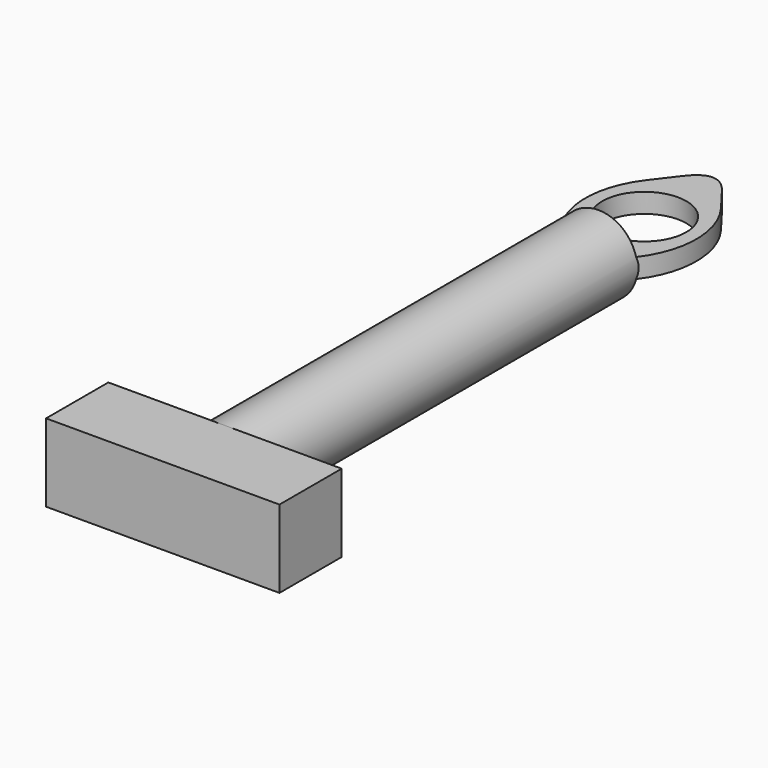
from build123d import *

# Parameters (mm, degrees)
F0_R        = 1.5875
F1_DEPTH    = 25.4
F2_W        = 9.525
F2_H        = 3.175
F3_DEPTH    = 3.175
F5_DEPTH    = 6.35
F7_DEPTH    = 25.4
F8_T1_DEPTH = 7.469008
F10_DEPTH   = 0.79375
F11_R       = 1.7145
F12_DEPTH   = 25.4


# Not quite as in the source:
# - a fillet or chamfer that OpenCascade refuses, or shapes differently, is made with other operations: its cross-section is extruded or revolved along the edge and cut away or added


with BuildPart() as f1:
    # F0 (on Front) → F1 (new body)
    with BuildSketch(Plane.XZ):
        Circle(F0_R)
    extrude(amount=F1_DEPTH)

    # F2 (on face) → F3 (join)
    with BuildSketch(Plane.XZ.offset(25.4)):
        Rectangle(F2_W, F2_H)
    extrude(amount=F3_DEPTH)

    # F4 (on face) → F5 (cut)
    with BuildSketch(Plane(origin=(0, 0, 0), x_dir=(-1, 0, 0), z_dir=(0, 1, 0))):
        with BuildLine():
            Line((-1.53709, 0.396875), (1.53709, 0.396875))
            ThreePointArc((1.53709, 0.396875), (0, 1.5875), (-1.53709, 0.396875))
        make_face()
        with BuildLine():
            Line((1.53709, -0.396875), (-1.53709, -0.396875))
            ThreePointArc((-1.53709, -0.396875), (0, -1.5875), (1.53709, -0.396875))
        make_face()
    extrude(amount=-F5_DEPTH, mode=Mode.SUBTRACT)

    # F6 (on face) → F7 (cut)
    with BuildSketch(Plane(origin=(0, 0, -0.396875), x_dir=(1, 0, 0), z_dir=(0, 0, -1))):
        Polygon((1.53709, 2.019778), (0, 0), (-1.53709, 2.019778), (-2.909934, 3.823732), (-2.909934, -0.784444), (2.909934, -0.784444), (2.909934, 3.823732), align=None)
    extrude(amount=-F7_DEPTH, mode=Mode.SUBTRACT)

    # F8: fillet of radius 1.016 on 1 edges, made by hand

    # F8_s2 → F8_t1 (cut)
    with BuildSketch(Plane.XY.offset(-3.734504)):
        with BuildLine():
            add(Edge.make_bspline(
                [(0.808504, -1.062396), (0, 0), (-0.808504, -1.062396)],
                knots=[0, 0, 0, 1, 1, 1], degree=2, weights=[1, 1, 1]))
            Line((-0.808504, -1.062396), (0, 0))
            Line((0, 0), (0.808504, -1.062396))
        make_face()
    extrude(amount=F8_T1_DEPTH, mode=Mode.SUBTRACT)

    # F9 (on face) → F10 (join)
    with BuildSketch(Plane(origin=(0, 0, -0.396875), x_dir=(1, 0, 0), z_dir=(0, 0, -1))):
        with BuildLine():
            Line((-1.53709, 2.019778), (-0.808504, 1.062396))
            add(Edge.make_bspline(
                [(-0.808504, 1.062396), (-0.269501, 0.354132), (0.269501, 0.354132), (0.808504, 1.062396)],
                knots=[0, 0, 0, 0, 1, 1, 1, 1], degree=3))
            Line((0.808504, 1.062396), (1.53709, 2.019778))
            ThreePointArc((1.53709, 2.019778), (2.267242, 4.184889), (1.53709, 6.35))
            Line((1.53709, 6.35), (-1.53709, 6.35))
            ThreePointArc((-1.53709, 6.35), (-2.267242, 4.184889), (-1.53709, 2.019778))
        make_face()
    extrude(amount=-F10_DEPTH)

    # F11 (on face) → F12 (cut)
    with BuildSketch(Plane(origin=(0, 0, -0.396875), x_dir=(1, 0, 0), z_dir=(0, 0, -1))):
        with Locations((0, 4.009057)):
            Circle(F11_R)
    extrude(amount=-F12_DEPTH, mode=Mode.SUBTRACT)


solid = f1.part
